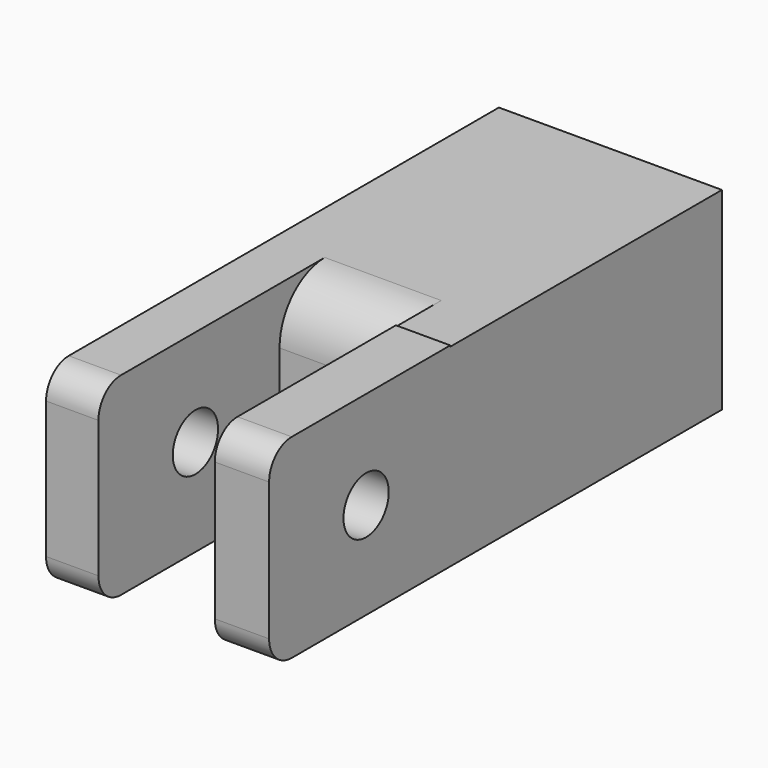
from build123d import *

# Parameters (mm, degrees)
F0_W     = 100.0908872011
F0_H     = 86.8150984859
F1_DEPTH = 152.4
F2_W     = 23.4895850481
F2_H     = 86.8150984859
F2_W_2   = 0.6694942713
F2_W_3   = 23.7127671899
F3_DEPTH = 101.6
F4_R     = 12.7
F6_D     = 25.4
F7_R     = 25.4


with BuildPart() as f1:
    # F0 (on Front) → F1 (new body)
    with BuildSketch(Plane.XZ):
        Rectangle(F0_W, F0_H)
    extrude(amount=F1_DEPTH)

    # F2 (on face) → F3 (join)
    with BuildSketch(Plane.XZ.offset(152.4)):
        with Locations((-38.3006510765, 0)):
            Rectangle(F2_W, F2_H)
        Polygon((25.6631821394, 43.9454764128), (25.6631821394, 43.4075492429), (26.3326764107, 43.4075492429), (50.0454436006, 43.4075492429), (50.0454436006, 43.9454764128), align=None)
        with Locations((25.997929275, 0)):
            Rectangle(F2_W_2, F2_H)
        with Locations((38.1890600056, 0)):
            Rectangle(F2_W_3, F2_H)
    extrude(amount=F3_DEPTH)

    # F4
    f4_edges = [f1.edges().sort_by_distance(p)[0] for p in [
        (-38.300651, -254, -43.407549),
        (37.854313, -254, -43.407549),
        (37.854313, -254, 43.945476),
        (-38.300651, -254, 43.407549),
    ]]
    fillet(f4_edges, radius=F4_R)

    # F6 (through all)
    with Locations(Plane(origin=(-50.0454436006, 0, 0), x_dir=(0, -1, 0), z_dir=(-1, 0, 0))):
        with Locations((199.5964795351, 0)):
            Hole(F6_D / 2)

    # F7
    f7_edges = [f1.edges().sort_by_distance(p)[0] for p in [
        (-0.446338, -152.4, -43.407549),
        (-0.446338, -152.4, 43.407549),
    ]]
    fillet(f7_edges, radius=F7_R)


solid = f1.part
